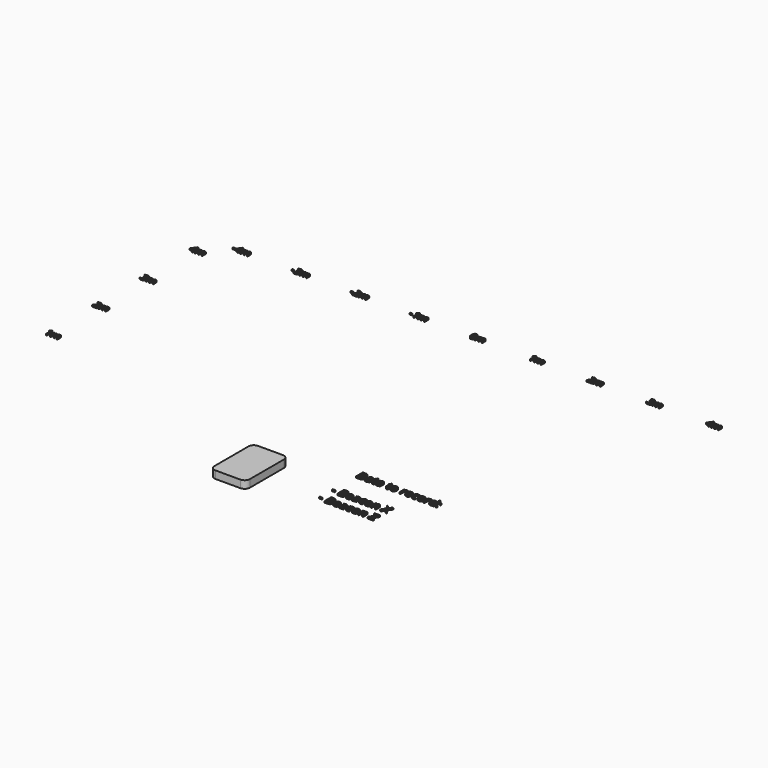
from build123d import *

# Parameters (mm, degrees)
F1_DEPTH     = 128
F3_TEXT_SIZE = 168.2793437106
F4_DEPTH     = 25
F5_TEXT_SIZE = 199.7624420456
F6_DEPTH     = 25


# Not quite as in the source:
# - Text() gives the source's letters only with a copy of the font that has no kerning and outlines rounded to 1/6400 em; it was checked with that copy


with BuildPart() as f1:
    # F0 (on Top) → F1 (new body)
    with BuildSketch(Plane.XY):
        with BuildLine():
            Line((210, 0), (-210, 0))
            ThreePointArc((-210, 0), (-273.6396103068, -26.3603896932), (-300, -90))
            Line((-300, -90), (-300, -810))
            ThreePointArc((-300, -810), (-273.6396103068, -873.6396103068), (-210, -900))
            Line((-210, -900), (210, -900))
            ThreePointArc((210, -900), (273.6396103068, -873.6396103068), (300, -810))
            Line((300, -810), (300, -90))
            ThreePointArc((300, -90), (273.6396103068, -26.3603896932), (210, 0))
        make_face()
    extrude(amount=F1_DEPTH)


with BuildPart() as f4:
    # F3 (on Top) → F4 (new body)
    with BuildSketch(Plane.XY):
        with Locations((-4574.9635268337, 911.8989442026)):
            Text('1m', F3_TEXT_SIZE, font='Open Sans', text_align=(TextAlign.LEFT, TextAlign.BOTTOM))
        with Locations((-4574.9635268337, 1934.7406303559)):
            Text('2m', F3_TEXT_SIZE, font='Open Sans', text_align=(TextAlign.LEFT, TextAlign.BOTTOM))
        with Locations((-4574.9635268337, 2937.1366178666)):
            Text('3m', F3_TEXT_SIZE, font='Open Sans', text_align=(TextAlign.LEFT, TextAlign.BOTTOM))
        with Locations((-4574.9635268337, 3976.2041246567)):
            Text('4m', F3_TEXT_SIZE, font='Open Sans', text_align=(TextAlign.LEFT, TextAlign.BOTTOM))
        with Locations((875, 4340.805863953)):
            Text('1m', F3_TEXT_SIZE, font='Open Sans', text_align=(TextAlign.LEFT, TextAlign.BOTTOM))
        with Locations((1875, 4340.805863953)):
            Text('2m', F3_TEXT_SIZE, font='Open Sans', text_align=(TextAlign.LEFT, TextAlign.BOTTOM))
        with Locations((2875, 4340.805863953)):
            Text('3m', F3_TEXT_SIZE, font='Open Sans', text_align=(TextAlign.LEFT, TextAlign.BOTTOM))
        with Locations((3875, 4340.805863953)):
            Text('4m', F3_TEXT_SIZE, font='Open Sans', text_align=(TextAlign.LEFT, TextAlign.BOTTOM))
        with Locations((-1152.0693100547, 4340.805863953)):
            Text('-1m', F3_TEXT_SIZE, font='Open Sans', text_align=(TextAlign.LEFT, TextAlign.BOTTOM))
        with Locations((-2152.0693100547, 4340.805863953)):
            Text('-2m', F3_TEXT_SIZE, font='Open Sans', text_align=(TextAlign.LEFT, TextAlign.BOTTOM))
        with Locations((-3152.0693100547, 4340.805863953)):
            Text('-3m', F3_TEXT_SIZE, font='Open Sans', text_align=(TextAlign.LEFT, TextAlign.BOTTOM))
        with Locations((-4152.0693100547, 4340.805863953)):
            Text('-4m', F3_TEXT_SIZE, font='Open Sans', text_align=(TextAlign.LEFT, TextAlign.BOTTOM))
        with Locations((-125, 4340.805863953)):
            Text('0m', F3_TEXT_SIZE, font='Open Sans', text_align=(TextAlign.LEFT, TextAlign.BOTTOM))
    extrude(amount=F4_DEPTH)


with BuildPart() as f6:
    # F5 (on Top) → F6 (new body)
    with BuildSketch(Plane.XY):
        with Locations((1203.2847731908, 285.6283131987)):
            Text('Data to record:', F5_TEXT_SIZE, font='Open Sans', text_align=(TextAlign.LEFT, TextAlign.BOTTOM))
        with Locations((1203.2847731908, -257.7255291654)):
            Text('- Beacon X', F5_TEXT_SIZE, font='Open Sans', text_align=(TextAlign.LEFT, TextAlign.BOTTOM))
        with Locations((1203.2847731908, -529.4024503475)):
            Text('- Beacon Z', F5_TEXT_SIZE, font='Open Sans', text_align=(TextAlign.LEFT, TextAlign.BOTTOM))
    extrude(amount=F6_DEPTH)


solid = Compound([f1.part, f4.part, f6.part])
